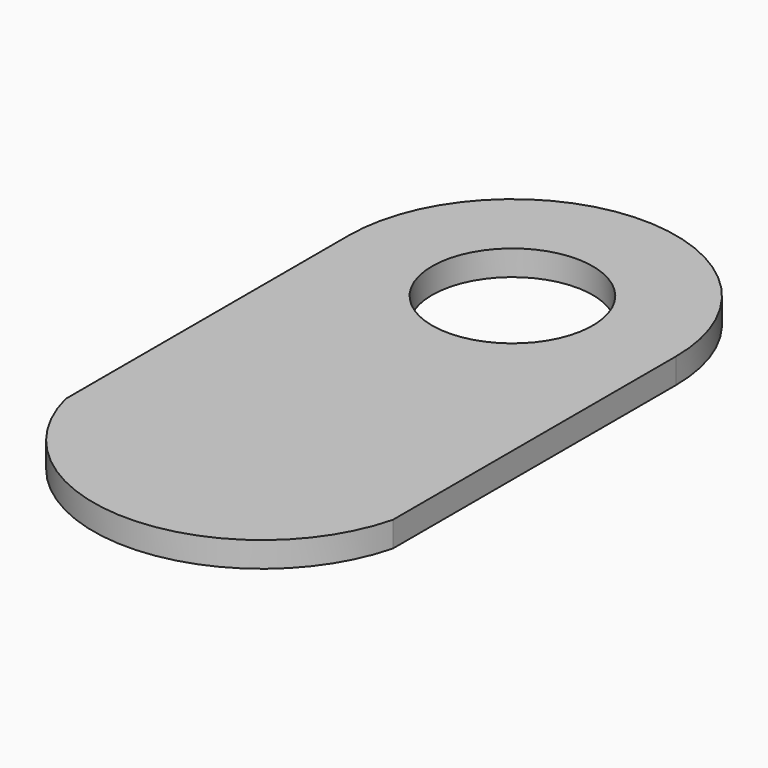
from build123d import *

# Parameters (mm, degrees)
F1_DEPTH = 2
F2_D     = 12.7


with BuildPart() as f1:
    # F0 (on Top) → F1 (new body)
    with BuildSketch(Plane.XY):
        with BuildLine():
            Line((-12.9365921021, 27.9824081808), (-12.9365921021, 0))
            ThreePointArc((-12.9365921021, 0), (0, -10.0852117819), (12.9365921021, 0))
            Line((12.9365921021, 0), (12.9365921021, 27.9824081808))
            ThreePointArc((12.9365921021, 27.9824081808), (0, 40.9190002829), (-12.9365921021, 27.9824081808))
        make_face()
    extrude(amount=F1_DEPTH)

    # F2 (through all)
    with Locations(Plane(origin=(0, 0, 0), x_dir=(1, 0, 0), z_dir=(0, 0, -1))):
        with Locations((0, -27.9824081808)):
            Hole(F2_D / 2)


solid = f1.part
